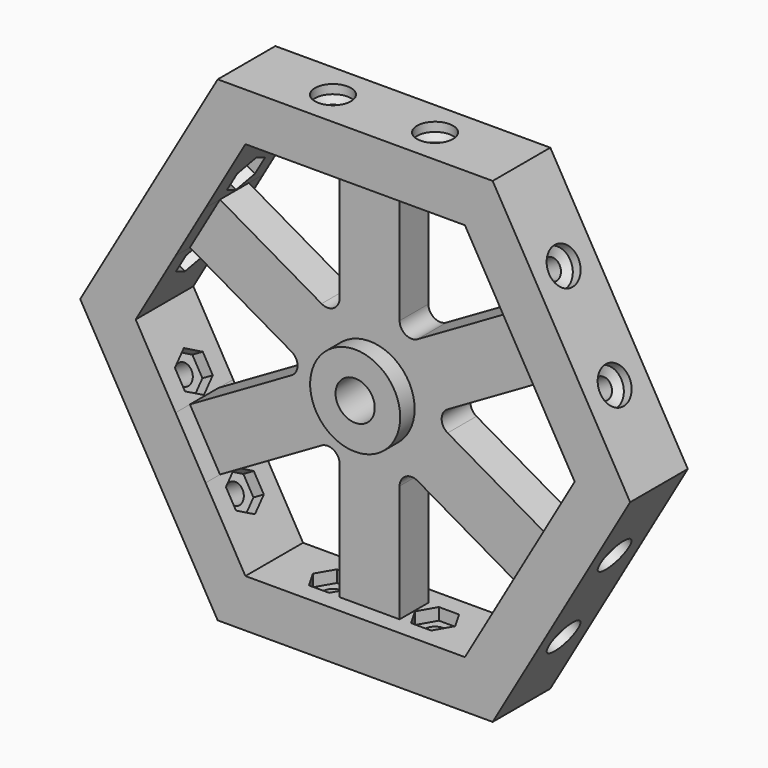
from build123d import *

# Parameters (mm, degrees)
F1_DEPTH  = 12
F2_START  = 3
F0_R      = 7.5
F0_R_2    = 5
F2_DEPTH  = 6
F4_START  = -6
F4_DEPTH  = 3
F5_D      = 3.3
F5_DEPTH  = 13.5
F5_TIP    = 0.9914200214
F6_D      = 6
F6_DEPTH  = 1.5
F6_TIP    = 1.8025818571
F7_DEPTH  = 12
F8_D      = 6.5278
F8_DEPTH  = 15.81
F8_TIP    = 1.9611489744
F10_START = -6
F10_DEPTH = 3
F11_D     = 6
F11_DEPTH = 1.5
F11_TIP   = 1.8025818571
F12_D     = 3.3
F12_DEPTH = 8
F12_START = 2.3111619
F12_TIP   = 0.9914200214
F14_START = -6
F14_DEPTH = 3
F15_D     = 3.3
F15_DEPTH = 8
F15_TIP   = 0.9914200214
F16_D     = 6
F16_DEPTH = 1.5
F16_TIP   = 1.8025818571
F18_START = -6
F18_DEPTH = 3
F19_D     = 6
F19_DEPTH = 1.5
F19_TIP   = 1.8025818571
F20_D     = 3.3
F20_DEPTH = 8
F20_START = 2.3111618
F20_TIP   = 0.9914200214
F22_START = -6
F22_DEPTH = 3
F23_D     = 3.3
F23_DEPTH = 8
F23_TIP   = 0.9914200214
F24_D     = 6
F24_DEPTH = 1.5
F24_TIP   = 1.8025818571
F26_START = -6
F26_DEPTH = 3
F27_D     = 6
F27_DEPTH = 1.5
F27_TIP   = 1.8025818571
F28_D     = 3.3
F28_DEPTH = 8
F28_START = 2.3111618
F28_TIP   = 0.9914200214


# Not quite as in the source:
# - a feature names something its author has since deleted; it is built from what else it names


with BuildPart() as f1:
    # F0 (on Front) → F1 (new body)
    with BuildSketch(Plane.XZ):
        Polygon((22.9, -39.6639634933), (45.8, 0), (22.9, 39.6639634933), (-22.9, 39.6639634933), (-45.8, 0), (-22.9, -39.6639634933), align=None)
        Polygon((29.9218283854, 11.5018729811), (36.5624378472, 0), (29.9218283854, -11.5018729811), (24.9218283854, -20.1621270189), (18.2812189236, -31.664), (5, -31.664), (-5, -31.664), (-18.2812189236, -31.664), (-24.9218283854, -20.1621270189), (-29.9218283854, -11.5018729811), (-36.5624378472, 0), (-29.9218283854, 11.5018729811), (-24.9218283854, 20.1621270189), (-18.2812189236, 31.664), (-5, 31.664), (5, 31.664), (18.2812189236, 31.664), (24.9218283854, 20.1621270189), align=None, mode=Mode.SUBTRACT)
    extrude(amount=F1_DEPTH)

    # F0 (on Front) → F2 (join)
    with BuildSketch(Plane.XZ.offset(F2_START)):
        with BuildLine():
            Line((24.9218283854, -20.1621270189), (29.9218283854, -11.5018729811))
            Line((29.9218283854, -11.5018729811), (13, -1.7320508076))
            ThreePointArc((13, -1.7320508076), (12, 0), (13, 1.7320508076))
            Line((13, 1.7320508076), (29.9218283854, 11.5018729811))
            Line((29.9218283854, 11.5018729811), (24.9218283854, 20.1621270189))
            Line((24.9218283854, 20.1621270189), (8, 10.3923048454))
            ThreePointArc((8, 10.3923048454), (6, 10.3923048454), (5, 12.124355653))
            Line((5, 12.124355653), (5, 31.664))
            Line((5, 31.664), (-5, 31.664))
            Line((-5, 31.664), (-5, 12.124355653))
            ThreePointArc((-5, 12.124355653), (-6, 10.3923048454), (-8, 10.3923048454))
            Line((-8, 10.3923048454), (-24.9218283854, 20.1621270189))
            Line((-24.9218283854, 20.1621270189), (-29.9218283854, 11.5018729811))
            Line((-29.9218283854, 11.5018729811), (-13, 1.7320508076))
            ThreePointArc((-13, 1.7320508076), (-12, 0), (-13, -1.7320508076))
            Line((-13, -1.7320508076), (-29.9218283854, -11.5018729811))
            Line((-29.9218283854, -11.5018729811), (-24.9218283854, -20.1621270189))
            Line((-24.9218283854, -20.1621270189), (-8, -10.3923048454))
            ThreePointArc((-8, -10.3923048454), (-6, -10.3923048454), (-5, -12.124355653))
            Line((-5, -12.124355653), (-5, -31.664))
            Line((-5, -31.664), (5, -31.664))
            Line((5, -31.664), (5, -12.124355653))
            ThreePointArc((5, -12.124355653), (6, -10.3923048454), (8, -10.3923048454))
            Line((8, -10.3923048454), (24.9218283854, -20.1621270189))
        make_face()
        Circle(F0_R, mode=Mode.SUBTRACT)
        Circle(F0_R)
        Circle(F0_R_2, mode=Mode.SUBTRACT)
        Circle(F0_R_2)
    extrude(amount=F2_DEPTH)

    # F3 (on face) → F4 (cut)
    with BuildSketch(Plane(origin=(-34.35, 0, -19.8319817467), x_dir=(0, -1, 0), z_dir=(-0.8660254038, 0, -0.5)).offset(F4_START)):
        Polygon((8.9, -6.8256842194), (6, -5.1513684387), (3.1, -6.8256842194), (3.1, -10.1743157806), (6, -11.8486315613), (8.9, -10.1743157806), align=None)
        Polygon((8.9, 6.8256842194), (8.9, 10.1743157806), (6, 11.8486315613), (3.1, 10.1743157806), (3.1, 6.8256842194), (6, 5.1513684387), align=None)
    extrude(amount=-F4_DEPTH, mode=Mode.SUBTRACT)

    # F5
    with Locations(Plane(origin=(-34.35, 0, -19.8319817467), x_dir=(0, -1, 0), z_dir=(-0.8660254038, 0, -0.5))):
        with Locations((6, -8.5), (6, 8.5)):
            Hole(F5_D / 2, depth=F5_DEPTH)
            with Locations((0, 0, -(F5_DEPTH + F5_TIP / 2))):  # 118° drill point
                Cone(0, F5_D / 2, F5_TIP, mode=Mode.SUBTRACT)

    # F6
    with Locations(Plane(origin=(-34.35, 0, -19.8319817467), x_dir=(0, -1, 0), z_dir=(-0.8660254038, 0, -0.5))):
        with Locations((6, -8.5), (6, 8.5)):
            Hole(F6_D / 2, depth=F6_DEPTH)
            with Locations((0, 0, -(F6_DEPTH + F6_TIP / 2))):  # 118° drill point
                Cone(0, F6_D / 2, F6_TIP, mode=Mode.SUBTRACT)

    # F0 (on Front) → F7 (join)
    with BuildSketch(Plane.XZ):
        Circle(F0_R)
        Circle(F0_R_2, mode=Mode.SUBTRACT)
        Circle(F0_R_2)
    extrude(amount=F7_DEPTH)

    # F8
    with Locations(Plane(origin=(0, 0, 0), x_dir=(1, 0, 0), z_dir=(0, 1, 0))):
        with Locations((0, 0)):
            Hole(F8_D / 2, depth=F8_DEPTH)
            with Locations((0, 0, -(F8_DEPTH + F8_TIP / 2))):  # 118° drill point
                Cone(0, F8_D / 2, F8_TIP, mode=Mode.SUBTRACT)

    # F9 (on face) → F10 (cut)
    with BuildSketch(Plane(origin=(-34.35, 0, 19.8319817467), x_dir=(0, -1, 0), z_dir=(-0.8660254038, 0, 0.5)).offset(F10_START)):
        Polygon((8.6710526316, -6.8256842194), (5.7710526316, -5.1513684387), (2.8710526316, -6.8256842194), (2.8710526316, -10.1743157806), (5.7710526316, -11.8486315613), (8.6710526316, -10.1743157806), align=None)
        Polygon((8.6710526316, 6.8256842194), (8.6710526316, 10.1743157806), (5.7710526316, 11.8486315613), (2.8710526316, 10.1743157806), (2.8710526316, 6.8256842194), (5.7710526316, 5.1513684387), align=None)
    extrude(amount=-F10_DEPTH, mode=Mode.SUBTRACT)

    # F11
    with Locations(Plane(origin=(-34.35, 0, 19.8319817467), x_dir=(0, -1, 0), z_dir=(-0.8660254038, 0, 0.5))):
        with Locations((5.7710526316, 8.5), (5.7710526316, -8.5)):
            Hole(F11_D / 2, depth=F11_DEPTH)
            with Locations((0, 0, -(F11_DEPTH + F11_TIP / 2))):  # 118° drill point
                Cone(0, F11_D / 2, F11_TIP, mode=Mode.SUBTRACT)

    # F12
    # its depths count from where the whole tool has entered the part; down to there all is cleared
    with Locations(Plane(origin=(-34.35, 0, 19.8319817467), x_dir=(0, -1, 0), z_dir=(-0.8660254038, 0, 0.5)).offset(-F12_START)):
        with Locations((5.7710526316, 8.5), (5.7710526316, -8.5)):
            Hole(F12_D / 2, depth=F12_DEPTH)
            with Locations((0, 0, -(F12_DEPTH + F12_TIP / 2))):  # 118° drill point
                Cone(0, F12_D / 2, F12_TIP, mode=Mode.SUBTRACT)

    # F13 (on face) → F14 (cut)
    with BuildSketch(Plane.XY.offset(39.6639634933).offset(F14_START)):
        Polygon((6.8256842194, -3.1), (5.1513684387, -6), (6.8256842194, -8.9), (10.1743157806, -8.9), (11.8486315613, -6), (10.1743157806, -3.1), align=None)
        Polygon((-10.1743157806, -3.1), (-11.8486315613, -6), (-10.1743157806, -8.9), (-6.8256842194, -8.9), (-5.1513684387, -6), (-6.8256842194, -3.1), align=None)
    extrude(amount=-F14_DEPTH, mode=Mode.SUBTRACT)

    # F15
    with Locations(Plane.XY.offset(39.6639634933)):
        with Locations((8.5, -6), (-8.5, -6)):
            Hole(F15_D / 2, depth=F15_DEPTH)
            with Locations((0, 0, -(F15_DEPTH + F15_TIP / 2))):  # 118° drill point
                Cone(0, F15_D / 2, F15_TIP, mode=Mode.SUBTRACT)

    # F16
    with Locations(Plane.XY.offset(39.6639634933)):
        with Locations((8.5, -6), (-8.5, -6)):
            Hole(F16_D / 2, depth=F16_DEPTH)
            with Locations((0, 0, -(F16_DEPTH + F16_TIP / 2))):  # 118° drill point
                Cone(0, F16_D / 2, F16_TIP, mode=Mode.SUBTRACT)

    # F17 (on face) → F18 (cut)
    with BuildSketch(Plane(origin=(34.35, 0, 19.8319817467), x_dir=(0, 1, 0), z_dir=(0.8660254038, 0, 0.5)).offset(F18_START)):
        Polygon((-3.3289473684, 6.8256842194), (-3.3289473684, 10.1743157806), (-6.2289473684, 11.8486315613), (-9.1289473684, 10.1743157806), (-9.1289473684, 6.8256842194), (-6.2289473684, 5.1513684387), align=None)
        Polygon((-3.3289473684, -6.8256842194), (-6.2289473684, -5.1513684387), (-9.1289473684, -6.8256842194), (-9.1289473684, -10.1743157806), (-6.2289473684, -11.8486315613), (-3.3289473684, -10.1743157806), align=None)
    extrude(amount=-F18_DEPTH, mode=Mode.SUBTRACT)

    # F19
    with Locations(Plane(origin=(34.35, 0, 19.8319817467), x_dir=(0, 1, 0), z_dir=(0.8660254038, 0, 0.5))):
        with Locations((-6.2289473684, -8.5), (-6.2289473684, 8.5)):
            Hole(F19_D / 2, depth=F19_DEPTH)
            with Locations((0, 0, -(F19_DEPTH + F19_TIP / 2))):  # 118° drill point
                Cone(0, F19_D / 2, F19_TIP, mode=Mode.SUBTRACT)

    # F20
    # its depths count from where the whole tool has entered the part; down to there all is cleared
    with Locations(Plane(origin=(34.35, 0, 19.8319817467), x_dir=(0, 1, 0), z_dir=(0.8660254038, 0, 0.5)).offset(-F20_START)):
        with Locations((-6.2289473684, -8.5), (-6.2289473684, 8.5)):
            Hole(F20_D / 2, depth=F20_DEPTH)
            with Locations((0, 0, -(F20_DEPTH + F20_TIP / 2))):  # 118° drill point
                Cone(0, F20_D / 2, F20_TIP, mode=Mode.SUBTRACT)

    # F21 (on face) → F22 (cut)
    with BuildSketch(Plane(origin=(34.35, 0, -19.8319817467), x_dir=(0, 1, 0), z_dir=(0.8660254038, 0, -0.5)).offset(F22_START)):
        Polygon((-3.3289473684, 6.8256842194), (-3.3289473684, 10.1743157806), (-6.2289473684, 11.8486315613), (-9.1289473684, 10.1743157806), (-9.1289473684, 6.8256842194), (-6.2289473684, 5.1513684387), align=None)
        Polygon((-3.3289473684, -6.8256842194), (-6.2289473684, -5.1513684387), (-9.1289473684, -6.8256842194), (-9.1289473684, -10.1743157806), (-6.2289473684, -11.8486315613), (-3.3289473684, -10.1743157806), align=None)
    extrude(amount=-F22_DEPTH, mode=Mode.SUBTRACT)

    # F23
    with Locations(Plane(origin=(34.35, 0, -19.8319817467), x_dir=(0, 1, 0), z_dir=(0.8660254038, 0, -0.5))):
        with Locations((-6.2289473684, -8.5), (-6.2289473684, 8.5)):
            Hole(F23_D / 2, depth=F23_DEPTH)
            with Locations((0, 0, -(F23_DEPTH + F23_TIP / 2))):  # 118° drill point
                Cone(0, F23_D / 2, F23_TIP, mode=Mode.SUBTRACT)

    # F24
    with Locations(Plane(origin=(34.35, 0, -19.8319817467), x_dir=(0, 1, 0), z_dir=(0.8660254038, 0, -0.5))):
        with Locations((-6.2289473684, -8.5), (-6.2289473684, 8.5)):
            Hole(F24_D / 2, depth=F24_DEPTH)
            with Locations((0, 0, -(F24_DEPTH + F24_TIP / 2))):  # 118° drill point
                Cone(0, F24_D / 2, F24_TIP, mode=Mode.SUBTRACT)

    # F25 (on face) → F26 (cut)
    with BuildSketch(Plane(origin=(0, 0, -39.6639634933), x_dir=(1, 0, 0), z_dir=(0, 0, -1)).offset(F26_START)):
        Polygon((-6.8256842194, 3.1), (-5.1513684387, 6), (-6.8256842194, 8.9), (-10.1743157806, 8.9), (-11.8486315613, 6), (-10.1743157806, 3.1), align=None)
        Polygon((6.8256842194, 3.1), (10.1743157806, 3.1), (11.8486315613, 6), (10.1743157806, 8.9), (6.8256842194, 8.9), (5.1513684387, 6), align=None)
    extrude(amount=-F26_DEPTH, mode=Mode.SUBTRACT)

    # F27
    with Locations(Plane(origin=(0, 0, -39.6639634933), x_dir=(1, 0, 0), z_dir=(0, 0, -1))):
        with Locations((-8.5, 6), (8.5, 6)):
            Hole(F27_D / 2, depth=F27_DEPTH)
            with Locations((0, 0, -(F27_DEPTH + F27_TIP / 2))):  # 118° drill point
                Cone(0, F27_D / 2, F27_TIP, mode=Mode.SUBTRACT)

    # F28
    # its depths count from where the whole tool has entered the part; down to there all is cleared
    with Locations(Plane(origin=(0, 0, -39.6639634933), x_dir=(1, 0, 0), z_dir=(0, 0, -1)).offset(-F28_START)):
        with Locations((-8.5, 6), (8.5, 6)):
            Hole(F28_D / 2, depth=F28_DEPTH)
            with Locations((0, 0, -(F28_DEPTH + F28_TIP / 2))):  # 118° drill point
                Cone(0, F28_D / 2, F28_TIP, mode=Mode.SUBTRACT)


solid = f1.part
